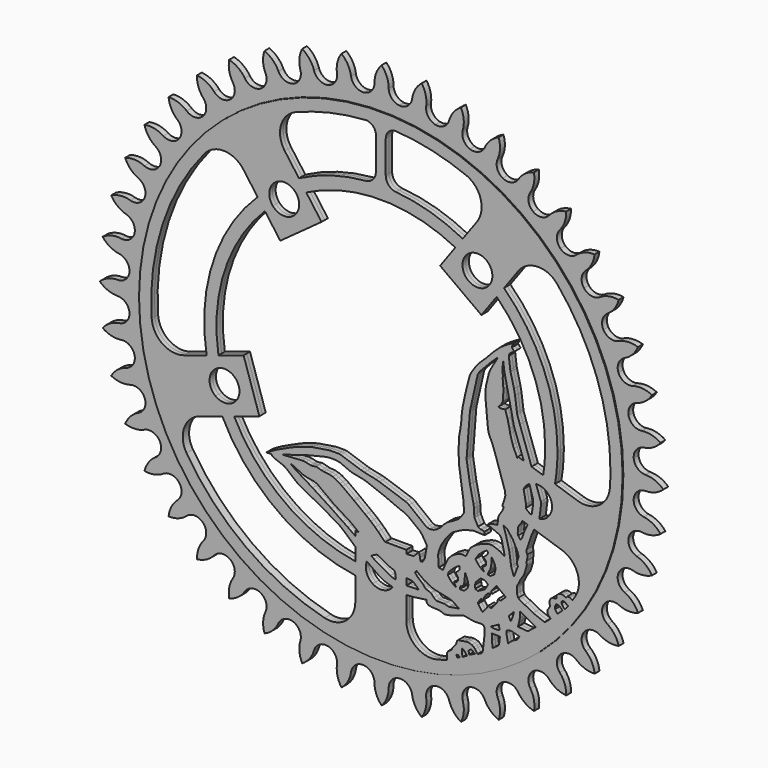
from build123d import *

# Parameters (mm, degrees)
F0_R     = 80.9142382347
F2_DEPTH = 1.016
F3_DEPTH = 1.3335


with BuildPart() as f2:
    # F0 (on Front) → F2 (new body, symmetric)
    with BuildSketch(Plane.XZ):
        with BuildLine():
            ThreePointArc((-2.3807027903, 88.3304793387), (-3.3502506643, 85.7312942415), (-5.785181868, 84.402047732))
            Line((-5.785181868, 84.402047732), (-5.784605012, 84.3980316838))
            ThreePointArc((-5.784605012, 84.3980316838), (-5.9092603745, 84.3841742706), (-6.0342913654, 84.3742627321))
            ThreePointArc((-6.0342913654, 84.3742627321), (-8.7897180441, 85.2562322534), (-10.2143039118, 87.7743270737))
            ThreePointArc((-10.2143039118, 87.7743270737), (-11.290613586, 90.8761740073), (-13.4364336422, 93.361199802))
            ThreePointArc((-13.4364336422, 93.361199802), (-14.7809344243, 90.3694083773), (-14.9266613405, 87.0926322257))
            ThreePointArc((-14.9266613405, 87.0926322257), (-15.585867257, 84.277565033), (-17.9800333254, 82.6567243326))
            ThreePointArc((-17.9800333254, 82.6567243326), (-20.8329310834, 83.1375785737), (-22.6013789781, 85.4273031122))
            ThreePointArc((-22.6013789781, 85.4273031122), (-24.1081722164, 88.3444028793), (-26.5858069626, 90.4987526602))
            ThreePointArc((-26.5858069626, 90.4987526602), (-27.4908463526, 87.346070947), (-27.1687561108, 84.0819085494))
            ThreePointArc((-27.1687561108, 84.0819085494), (-27.4206264293, 81.2016798984), (-29.5597536571, 79.2566116624))
            ThreePointArc((-29.5597536571, 79.2566116624), (-32.452045723, 79.3265618177), (-34.5283551454, 81.3413038857))
            ThreePointArc((-34.5283551454, 81.3413038857), (-36.4349579827, 84.0142727472), (-39.1939699203, 85.7940901655))
            ThreePointArc((-39.1939699203, 85.7940901655), (-39.6411239261, 82.544697672), (-38.8577733549, 79.3595979617))
            ThreePointArc((-38.8577733549, 79.3595979617), (-38.697180722, 76.4728410018), (-40.5377226476, 74.2431412103))
            ThreePointArc((-40.5377226476, 74.2431412103), (-43.4105302956, 73.9007632963), (-45.7524335735, 75.5995085554))
            ThreePointArc((-45.7524335735, 75.5995085554), (-48.0200330743, 77.9739325737), (-51.0042566765, 79.3429856792))
            ThreePointArc((-51.0042566765, 79.3429856792), (-50.9844225321, 76.063030666), (-49.7557583901, 73.0218330881))
            ThreePointArc((-49.7557583901, 73.0218330881), (-49.1859720087, 70.1873138662), (-50.6904605062, 67.7183727772))
            ThreePointArc((-50.6904605062, 67.7183727772), (-53.4853016571, 66.9706366209), (-56.0451243932, 68.3188035164))
            ThreePointArc((-56.0451243932, 68.3188035164), (-58.6275587708, 70.3463462656), (-61.776243851, 71.2767650851))
            ThreePointArc((-61.776243851, 71.2767650851), (-61.2898253223, 68.0330179777), (-59.6408596681, 65.1976325448))
            ThreePointArc((-59.6408596681, 65.1976325448), (-58.673478746, 62.4730536983), (-59.811286768, 59.8151318325))
            ThreePointArc((-59.811286768, 59.8151318325), (-62.4712665157, 58.6772591857), (-65.196898101, 59.6474029274))
            ThreePointArc((-65.196898101, 59.6474029274), (-68.0415964386, 61.286789484), (-71.2906448486, 61.7596333736))
            ThreePointArc((-71.2906448486, 61.7596333736), (-70.3475440142, 58.6181275089), (-68.3118450334, 56.0462744918))
            ThreePointArc((-68.3118450334, 56.0462744918), (-66.9665626563, 53.4871005889), (-67.7145277128, 50.6943055706))
            ThreePointArc((-67.7145277128, 50.6943055706), (-70.1854965403, 49.1894602391), (-73.0214509758, 49.7618314981))
            ThreePointArc((-73.0214509758, 49.7618314981), (-76.0705034187, 50.9796886795), (-79.3537739023, 50.9853319011))
            ThreePointArc((-79.3537739023, 50.9853319011), (-77.9731895755, 48.0100192791), (-75.5921982289, 45.7540541887))
            ThreePointArc((-75.5921982289, 45.7540541887), (-73.8964004665, 43.41238263), (-74.2392961459, 40.5415677121))
            ThreePointArc((-74.2392961459, 40.5415677121), (-76.4709522536, 38.7003840072), (-79.3594976852, 38.8633309552))
            ThreePointArc((-79.3594976852, 38.8633309552), (-82.5508343185, 39.6348667012), (-85.8014889567, 39.1731943751))
            ThreePointArc((-85.8014889567, 39.1731943751), (-84.0115258531, 36.4246437807), (-81.3337122584, 34.5304915605))
            ThreePointArc((-81.3337122584, 34.5304915605), (-79.3219206629, 32.4539920261), (-79.2527665979, 29.5635987216))
            ThreePointArc((-79.2527665979, 29.5635987216), (-81.199679903, 27.423557834), (-84.0820138756, 27.1737633411))
            ThreePointArc((-84.0820138756, 27.1737633411), (-87.3506682884, 27.4832714088), (-90.5025331271, 26.5636818521))
            ThreePointArc((-90.5025331271, 26.5636818521), (-88.3396297336, 24.0978458494), (-85.4195064533, 22.6040659762))
            ThreePointArc((-85.4195064533, 22.6040659762), (-83.1326753001, 20.8350100086), (-82.6528792681, 17.9838783899))
            ThreePointArc((-82.6528792681, 17.9838783899), (-84.2754162302, 15.5885453807), (-87.0928627361, 14.9310945424))
            ThreePointArc((-87.0928627361, 14.9310945424), (-90.3722945505, 14.7722742402), (-93.3612067107, 13.4134876445))
            ThreePointArc((-93.3612067107, 13.4134876445), (-90.8693935032, 11.2805635434), (-87.7664058264, 10.2175650679))
            ThreePointArc((-87.7664058264, 10.2175650679), (-85.2510884031, 8.791965545), (-84.3704176676, 6.0381364299))
            ThreePointArc((-84.3704176676, 6.0381364299), (-85.6355481131, 3.4362733715), (-88.3307520663, 2.384549991))
            ThreePointArc((-88.3307520663, 2.384549991), (-91.5542015078, 1.7606344421), (-94.3193153572, -0.0096882159))
            ThreePointArc((-94.3193153572, -0.0096882159), (-91.5493184668, -1.7662802314), (-88.3266342742, -2.3768577258))
            ThreePointArc((-88.3266342742, -2.3768577258), (-85.6340351899, -3.4299797088), (-84.3704176676, -6.0304463009))
            ThreePointArc((-84.3704176676, -6.0304463009), (-85.252387189, -8.7858729796), (-87.7704820093, -10.2104588474))
            ThreePointArc((-87.7704820093, -10.2104588474), (-90.8723289428, -11.2867685215), (-93.3573547375, -13.4325885778))
            ThreePointArc((-93.3573547375, -13.4325885778), (-90.3655633128, -14.7770893599), (-87.0887871612, -14.922816276))
            ThreePointArc((-87.0887871612, -14.922816276), (-84.2737199685, -15.5820221925), (-82.6528792681, -17.976188261))
            ThreePointArc((-82.6528792681, -17.976188261), (-83.1337335093, -20.8290860189), (-85.4234580477, -22.5975339137))
            ThreePointArc((-85.4234580477, -22.5975339137), (-88.3405578148, -24.1043271519), (-90.4949075957, -26.5819618981))
            ThreePointArc((-90.4949075957, -26.5819618981), (-87.3422258826, -27.4870012881), (-84.078063485, -27.1649110463))
            ThreePointArc((-84.078063485, -27.1649110463), (-81.1978348339, -27.4167813648), (-79.2527665979, -29.5559085926))
            ThreePointArc((-79.2527665979, -29.5559085926), (-79.3227167532, -32.4482006585), (-81.3374588212, -34.524510081))
            ThreePointArc((-81.3374588212, -34.524510081), (-84.0104276828, -36.4311129182), (-85.790245101, -39.1901248558))
            ThreePointArc((-85.790245101, -39.1901248558), (-82.5408526075, -39.6372788617), (-79.3557528972, -38.8539282904))
            ThreePointArc((-79.3557528972, -38.8539282904), (-76.4689959373, -38.6933356575), (-74.2392961459, -40.5338775831))
            ThreePointArc((-74.2392961459, -40.5338775831), (-73.8969182319, -43.4066852311), (-75.595663491, -45.7485885091))
            ThreePointArc((-75.595663491, -45.7485885091), (-77.9700875092, -48.0161880098), (-79.3391406147, -51.0004116121))
            ThreePointArc((-79.3391406147, -51.0004116121), (-76.0591856015, -50.9805774677), (-73.0179880236, -49.7519133256))
            ThreePointArc((-73.0179880236, -49.7519133256), (-70.1834688017, -49.1821269442), (-67.7145277128, -50.6866154417))
            ThreePointArc((-67.7145277128, -50.6866154417), (-66.9667915564, -53.4814565926), (-68.3149584519, -56.0412793287))
            ThreePointArc((-68.3149584519, -56.0412793287), (-70.3425012011, -58.6237137063), (-71.2729200207, -61.7723987865))
            ThreePointArc((-71.2729200207, -61.7723987865), (-68.0291729133, -61.2859802578), (-65.1937874804, -59.6370146037))
            ThreePointArc((-65.1937874804, -59.6370146037), (-62.4692086338, -58.6696336815), (-59.811286768, -59.8074417035))
            ThreePointArc((-59.811286768, -59.8074417035), (-58.6734141212, -62.4674214512), (-59.6435578629, -65.1930530365))
            ThreePointArc((-59.6435578629, -65.1930530365), (-61.2829444195, -68.0377513741), (-61.7557883091, -71.2867997841))
            ThreePointArc((-61.7557883091, -71.2867997841), (-58.6142824444, -70.3436989497), (-56.0424294273, -68.307999969))
            ThreePointArc((-56.0424294273, -68.307999969), (-53.4832555244, -66.9627175918), (-50.6904605062, -67.7106826483))
            ThreePointArc((-50.6904605062, -67.7106826483), (-49.1856151746, -70.1816514758), (-49.7579864336, -73.0176059113))
            ThreePointArc((-49.7579864336, -73.0176059113), (-50.975843615, -76.0666583542), (-50.9814868366, -79.3499288378))
            ThreePointArc((-50.9814868366, -79.3499288378), (-48.0061742147, -77.969344511), (-45.7502091242, -75.5883531645))
            ThreePointArc((-45.7502091242, -75.5883531645), (-43.4085375655, -73.8925554021), (-40.5377226476, -74.2354510814))
            ThreePointArc((-40.5377226476, -74.2354510814), (-38.6965389427, -76.4671071891), (-38.8594858907, -79.3556526207))
            ThreePointArc((-38.8594858907, -79.3556526207), (-39.6310216367, -82.546989254), (-39.1693493106, -85.7976438922))
            ThreePointArc((-39.1693493106, -85.7976438922), (-36.4207987163, -84.0076807886), (-34.526646496, -81.3298671939))
            ThreePointArc((-34.526646496, -81.3298671939), (-32.4501469617, -79.3180755984), (-29.5597536571, -79.2489215334))
            ThreePointArc((-29.5597536571, -79.2489215334), (-27.4197127695, -81.1958348385), (-27.1699182766, -84.0781688112))
            ThreePointArc((-27.1699182766, -84.0781688112), (-27.4794263443, -87.3468232239), (-26.5598367877, -90.4986880626))
            ThreePointArc((-26.5598367877, -90.4986880626), (-24.0940007849, -88.3357846692), (-22.6002209117, -85.4156613888))
            ThreePointArc((-22.6002209117, -85.4156613888), (-20.8311649442, -83.1288302356), (-17.9800333254, -82.6490342036))
            ThreePointArc((-17.9800333254, -82.6490342036), (-15.5847003162, -84.2715711657), (-14.9272494779, -87.0890176716))
            ThreePointArc((-14.9272494779, -87.0890176716), (-14.7684291757, -90.368449486), (-13.40964258, -93.3573616462))
            ThreePointArc((-13.40964258, -93.3573616462), (-11.2767184789, -90.8655484388), (-10.2137200034, -87.7625607619))
            ThreePointArc((-10.2137200034, -87.7625607619), (-8.7881204805, -85.2472433386), (-6.0342913654, -84.3665726031))
            ThreePointArc((-6.0342913654, -84.3665726031), (-3.4324283071, -85.6317030486), (-2.3807049265, -88.3269070018))
            ThreePointArc((-2.3807049265, -88.3269070018), (-1.7567893776, -91.5503564433), (0.0135332804, -94.3154702927))
            ThreePointArc((0.0135332804, -94.3154702927), (1.7701252959, -91.5454734023), (2.3807027903, -88.3227892097))
            ThreePointArc((2.3807027903, -88.3227892097), (3.4338247732, -85.6301901255), (6.0342913654, -84.3665726031))
            ThreePointArc((6.0342913654, -84.3665726031), (8.7897180441, -85.2485421245), (10.2143039118, -87.7666369448))
            ThreePointArc((10.2143039118, -87.7666369448), (11.290613586, -90.8684838784), (13.4364336422, -93.353509673))
            ThreePointArc((13.4364336422, -93.353509673), (14.7809344243, -90.3617182483), (14.9266613405, -87.0849420968))
            ThreePointArc((14.9266613405, -87.0849420968), (15.585867257, -84.2698749041), (17.9800333254, -82.6490342036))
            ThreePointArc((17.9800333254, -82.6490342036), (20.8329310834, -83.1298884448), (22.6013789781, -85.4196129832))
            ThreePointArc((22.6013789781, -85.4196129832), (24.1081722164, -88.3367127503), (26.5858069626, -90.4910625312))
            ThreePointArc((26.5858069626, -90.4910625312), (27.4908463526, -87.3383808181), (27.1687561108, -84.0742184205))
            ThreePointArc((27.1687561108, -84.0742184205), (27.4206264293, -81.1939897694), (29.5597536571, -79.2489215334))
            ThreePointArc((29.5597536571, -79.2489215334), (32.452045723, -79.3188716887), (34.5283551454, -81.3336137567))
            ThreePointArc((34.5283551454, -81.3336137567), (36.4349579827, -84.0065826183), (39.1939699203, -85.7864000365))
            ThreePointArc((39.1939699203, -85.7864000365), (39.6411239261, -82.537007543), (38.8577733549, -79.3519078328))
            ThreePointArc((38.8577733549, -79.3519078328), (38.697180722, -76.4651508728), (40.5377226476, -74.2354510814))
            ThreePointArc((40.5377226476, -74.2354510814), (43.4105302956, -73.8930731674), (45.7524335735, -75.5918184265))
            ThreePointArc((45.7524335735, -75.5918184265), (48.0200330743, -77.9662424447), (51.0042566765, -79.3352955502))
            ThreePointArc((51.0042566765, -79.3352955502), (50.9844225321, -76.055340537), (49.7557583901, -73.0141429592))
            ThreePointArc((49.7557583901, -73.0141429592), (49.1859720087, -70.1796237372), (50.6904605062, -67.7106826483))
            ThreePointArc((50.6904605062, -67.7106826483), (53.4853016571, -66.962946492), (56.0451243932, -68.3111133875))
            ThreePointArc((56.0451243932, -68.3111133875), (58.6275587708, -70.3386561366), (61.776243851, -71.2690749562))
            ThreePointArc((61.776243851, -71.2690749562), (61.2898253223, -68.0253278488), (59.6408596681, -65.1899424159))
            ThreePointArc((59.6408596681, -65.1899424159), (58.673478746, -62.4653635693), (59.811286768, -59.8074417035))
            ThreePointArc((59.811286768, -59.8074417035), (62.4712665157, -58.6695690567), (65.196898101, -59.6397127984))
            ThreePointArc((65.196898101, -59.6397127984), (68.0415964386, -61.2790993551), (71.2906448486, -61.7519432447))
            ThreePointArc((71.2906448486, -61.7519432447), (70.3475440142, -58.61043738), (68.3118450334, -56.0385843628))
            ThreePointArc((68.3118450334, -56.0385843628), (66.9665626563, -53.4794104599), (67.7145277128, -50.6866154417))
            ThreePointArc((67.7145277128, -50.6866154417), (70.1854965403, -49.1817701101), (73.0214509758, -49.7541413691))
            ThreePointArc((73.0214509758, -49.7541413691), (76.0705034187, -50.9719985506), (79.3537739023, -50.9776417721))
            ThreePointArc((79.3537739023, -50.9776417721), (77.9731895755, -48.0023291502), (75.5921982289, -45.7463640597))
            ThreePointArc((75.5921982289, -45.7463640597), (73.8964004665, -43.404692501), (74.2392961459, -40.5338775831))
            ThreePointArc((74.2392961459, -40.5338775831), (76.4709522536, -38.6926938782), (79.3594976852, -38.8556408262))
            ThreePointArc((79.3594976852, -38.8556408262), (82.5508343185, -39.6271765723), (85.8014889567, -39.1655042461))
            ThreePointArc((85.8014889567, -39.1655042461), (84.0115258531, -36.4169536518), (81.3337122584, -34.5228014315))
            ThreePointArc((81.3337122584, -34.5228014315), (79.3219206629, -32.4463018972), (79.2527665979, -29.5559085926))
            ThreePointArc((79.2527665979, -29.5559085926), (81.199679903, -27.415867705), (84.0820138756, -27.1660732121))
            ThreePointArc((84.0820138756, -27.1660732121), (87.3506682884, -27.4755812799), (90.5025331271, -26.5559917232))
            ThreePointArc((90.5025331271, -26.5559917232), (88.3396297336, -24.0901557204), (85.4195064533, -22.5963758473))
            ThreePointArc((85.4195064533, -22.5963758473), (83.1326753001, -20.8273198797), (82.6528792681, -17.976188261))
            ThreePointArc((82.6528792681, -17.976188261), (84.2754162302, -15.5808552517), (87.0928627361, -14.9234044134))
            ThreePointArc((87.0928627361, -14.9234044134), (90.3722945505, -14.7645841112), (93.3612067107, -13.4057975155))
            ThreePointArc((93.3612067107, -13.4057975155), (90.8693935032, -11.2728734145), (87.7664058264, -10.2098749389))
            ThreePointArc((87.7664058264, -10.2098749389), (85.2510884031, -8.7842754161), (84.3704176676, -6.0304463009))
            ThreePointArc((84.3704176676, -6.0304463009), (85.6355481131, -3.4285832426), (88.3307520663, -2.376859862))
            ThreePointArc((88.3307520663, -2.376859862), (91.5542015078, -1.7529443132), (94.3193153572, 0.0173783449))
            ThreePointArc((94.3193153572, 0.0173783449), (91.5493184668, 1.7739703604), (88.3266342742, 2.3845478548))
            ThreePointArc((88.3266342742, 2.3845478548), (85.6340351899, 3.4376698377), (84.3704176676, 6.0381364299))
            ThreePointArc((84.3704176676, 6.0381364299), (85.252387189, 8.7935631086), (87.7704820093, 10.2181489763))
            ThreePointArc((87.7704820093, 10.2181489763), (90.8723289428, 11.2944586504), (93.3573547375, 13.4402787067))
            ThreePointArc((93.3573547375, 13.4402787067), (90.3655633128, 14.7847794888), (87.0887871612, 14.930506405))
            ThreePointArc((87.0887871612, 14.930506405), (84.2737199685, 15.5897123214), (82.6528792681, 17.9838783899))
            ThreePointArc((82.6528792681, 17.9838783899), (83.1337335093, 20.8367761478), (85.4234580477, 22.6052240426))
            ThreePointArc((85.4234580477, 22.6052240426), (88.3405578148, 24.1120172809), (90.4949075957, 26.5896520271))
            ThreePointArc((90.4949075957, 26.5896520271), (87.3422258826, 27.4946914171), (84.078063485, 27.1726011753))
            ThreePointArc((84.078063485, 27.1726011753), (81.1978348339, 27.4244714937), (79.2527665979, 29.5635987216))
            ThreePointArc((79.2527665979, 29.5635987216), (79.3227167532, 32.4558907874), (81.3374588212, 34.5322002099))
            ThreePointArc((81.3374588212, 34.5322002099), (84.0104276828, 36.4388030472), (85.790245101, 39.1978149848))
            ThreePointArc((85.790245101, 39.1978149848), (82.5408526075, 39.6449689906), (79.3557528972, 38.8616184194))
            ThreePointArc((79.3557528972, 38.8616184194), (76.4689959373, 38.7010257865), (74.2392961459, 40.5415677121))
            ThreePointArc((74.2392961459, 40.5415677121), (73.8969182319, 43.4143753601), (75.595663491, 45.756278638))
            ThreePointArc((75.595663491, 45.756278638), (77.9700875092, 48.0238781388), (79.3391406147, 51.008101741))
            ThreePointArc((79.3391406147, 51.008101741), (76.0591856015, 50.9882675966), (73.0179880236, 49.7596034545))
            ThreePointArc((73.0179880236, 49.7596034545), (70.1834688017, 49.1898170732), (67.7145277128, 50.6943055706))
            ThreePointArc((67.7145277128, 50.6943055706), (66.9667915564, 53.4891467216), (68.3149584519, 56.0489694577))
            ThreePointArc((68.3149584519, 56.0489694577), (70.3425012011, 58.6314038353), (71.2729200207, 61.7800889154))
            ThreePointArc((71.2729200207, 61.7800889154), (68.0291729133, 61.2936703868), (65.1937874804, 59.6447047326))
            ThreePointArc((65.1937874804, 59.6447047326), (62.4692086338, 58.6773238104), (59.811286768, 59.8151318325))
            ThreePointArc((59.811286768, 59.8151318325), (58.6734141212, 62.4751115802), (59.6435578629, 65.2007431655))
            ThreePointArc((59.6435578629, 65.2007431655), (61.2829444195, 68.0454415031), (61.7557883091, 71.294489913))
            ThreePointArc((61.7557883091, 71.294489913), (58.6142824444, 70.3513890786), (56.0424294273, 68.3156900979))
            ThreePointArc((56.0424294273, 68.3156900979), (53.4832555244, 66.9704077208), (50.6904605062, 67.7183727772))
            ThreePointArc((50.6904605062, 67.7183727772), (49.1856151746, 70.1893416048), (49.7579864336, 73.0252960403))
            ThreePointArc((49.7579864336, 73.0252960403), (50.975843615, 76.0743484832), (50.9814868366, 79.3576189668))
            ThreePointArc((50.9814868366, 79.3576189668), (48.0061742147, 77.97703464), (45.7502091242, 75.5960432934))
            ThreePointArc((45.7502091242, 75.5960432934), (43.4085375655, 73.900245531), (40.5377226476, 74.2431412103))
            ThreePointArc((40.5377226476, 74.2431412103), (38.6965389427, 76.4747973181), (38.8594858907, 79.3633427497))
            ThreePointArc((38.8594858907, 79.3633427497), (39.6310216367, 82.5546793829), (39.1693493106, 85.8053340212))
            ThreePointArc((39.1693493106, 85.8053340212), (36.4207987163, 84.0153709176), (34.526646496, 81.3375573229))
            ThreePointArc((34.526646496, 81.3375573229), (32.4501469617, 79.3257657274), (29.5597536571, 79.2566116624))
            ThreePointArc((29.5597536571, 79.2566116624), (27.4197127695, 81.2035249675), (27.1699182766, 84.0858589401))
            ThreePointArc((27.1699182766, 84.0858589401), (27.4794263443, 87.3545133529), (26.5598367877, 90.5063781916))
            ThreePointArc((26.5598367877, 90.5063781916), (24.0940007849, 88.3434747981), (22.6002209117, 85.4233515178))
            ThreePointArc((22.6002209117, 85.4233515178), (20.8311649442, 83.1365203646), (17.9800333254, 82.6567243326))
            ThreePointArc((17.9800333254, 82.6567243326), (15.5847003162, 84.2792612946), (14.9272494779, 87.0967078006))
            ThreePointArc((14.9272494779, 87.0967078006), (14.7684291757, 90.376139615), (13.40964258, 93.3650517752))
            ThreePointArc((13.40964258, 93.3650517752), (11.2767184789, 90.8732385677), (10.2137200034, 87.7702508909))
            ThreePointArc((10.2137200034, 87.7702508909), (8.7881204805, 85.2549334675), (6.0342913654, 84.3742627321))
            ThreePointArc((6.0342913654, 84.3742627321), (5.9092603745, 84.3841742706), (5.784605012, 84.3980316838))
            Line((5.784605012, 84.3980316838), (5.785181868, 84.402047732))
            ThreePointArc((5.785181868, 84.402047732), (3.3489026704, 85.7328505084), (2.3807049265, 88.3345971308))
            ThreePointArc((2.3807049265, 88.3345971308), (1.7567893776, 91.5580465723), (-0.0135332804, 94.3231604217))
            ThreePointArc((-0.0135332804, 94.3231604217), (-1.7701252959, 91.5531635313), (-2.3807027903, 88.3304793387))
        make_face()
        with Locations((0, -0.1371763303)):
            Circle(F0_R, mode=Mode.SUBTRACT)
    extrude(amount=F2_DEPTH, both=True)

    # F0 (on Front) + F1 (on Front) → F3 (join, symmetric)
    with BuildSketch(Plane.XZ):
        with Locations((0, -0.1371763303)):
            Circle(F0_R)
        with BuildLine():
            ThreePointArc((59.0317664993, 49.1858312889), (72.2472248739, 26.1563922256), (76.835, 0.0038450645))
            ThreePointArc((76.835, 0.0038450645), (76.7927755196, -2.5430850483), (76.666148487, -5.0872158431))
            ThreePointArc((76.666148487, -5.0872158431), (73.0744274295, -23.7394756983), (65.0166675393, -40.9406315726))
            ThreePointArc((65.0166675393, -40.9406315726), (45.1624798599, -62.1569756983), (18.8492561247, -74.4832193732))
            ThreePointArc((18.8492561247, -74.4832193732), (0, -76.8311549355), (-18.8492561247, -74.4832193732))
            ThreePointArc((-18.8492561247, -74.4832193732), (-45.1624798599, -62.1569756983), (-65.0166675393, -40.9406315726))
            ThreePointArc((-65.0166675393, -40.9406315726), (-73.0744274295, -23.7394756983), (-76.666148487, -5.0872158431))
            ThreePointArc((-76.666148487, -5.0872158431), (-73.0744274295, 23.7471658273), (-59.0317664993, 49.1858312889))
            ThreePointArc((-59.0317664993, 49.1858312889), (-45.1624798599, 62.1646658273), (-28.5330294268, 71.3444608225))
            ThreePointArc((-28.5330294268, 71.3444608225), (-17.0590244353, 74.9211789086), (-5.1676308023, 76.6648704743))
            ThreePointArc((-5.1676308023, 76.6648704743), (0, 76.8388450645), (5.1676308023, 76.6648704743))
            ThreePointArc((5.1676308023, 76.6648704743), (17.0590244353, 74.9211789086), (28.5330294268, 71.3444608225))
            ThreePointArc((28.5330294268, 71.3444608225), (45.1624798599, 62.1646658273), (59.0317664993, 49.1858312889))
        make_face(mode=Mode.SUBTRACT)
        with BuildLine():
            ThreePointArc((-76.666148487, -5.0872158431), (-73.0744274295, -23.7394756983), (-65.0166675393, -40.9406315726))
            ThreePointArc((-65.0166675393, -40.9406315726), (-65.7958321334, -33.7102587401), (-60.5690531989, -28.653958637))
            Line((-60.5690531989, -28.653958637), (-53.0574761233, -26.2132992954))
            ThreePointArc((-53.0574761233, -26.2132992954), (-54.2531303783, -23.6245730703), (-55.3225672779, -20.9812045218))
            ThreePointArc((-55.3225672779, -20.9812045218), (-57.067147534, -18.5255649228), (-57.0844390827, -15.5133519302))
            ThreePointArc((-57.0844390827, -15.5133519302), (-57.7576015726, -12.7514310465), (-58.2972156627, -9.9603432049))
            Line((-58.2972156627, -9.9603432049), (-65.84602775, -12.4131009352))
            ThreePointArc((-65.84602775, -12.4131009352), (-73.0465993656, -11.3946917979), (-76.666148487, -5.0872158431))
        make_face()
        with BuildLine():
            ThreePointArc((-32.1567589923, 58.7900914961), (-33.4132933444, 65.9529477828), (-28.5330294268, 71.3444608225))
            ThreePointArc((-28.5330294268, 71.3444608225), (-45.1624798599, 62.1646658273), (-59.0317664993, 49.1858312889))
            ThreePointArc((-59.0317664993, 49.1858312889), (-52.3960484026, 52.1611689343), (-45.9720577247, 48.7526894299))
            Line((-45.9720577247, 48.7526894299), (-41.232635647, 42.2294345687))
            ThreePointArc((-41.232635647, 42.2294345687), (-39.228199606, 44.0918674886), (-37.1397367415, 45.8595617741))
            ThreePointArc((-37.1397367415, 45.8595617741), (-35.2610281077, 48.5492802232), (-32.1195407916, 49.4954244559))
            ThreePointArc((-32.1195407916, 49.4954244559), (-29.7931161901, 50.9258258254), (-27.4031144293, 52.2472610633))
            Line((-27.4031144293, 52.2472610633), (-32.1567589923, 58.7900914961))
        make_face()
        with BuildLine():
            ThreePointArc((45.9720577247, 48.7526894299), (52.3960484026, 52.1611689343), (59.0317664993, 49.1858312889))
            ThreePointArc((59.0317664993, 49.1858312889), (45.1624798599, 62.1646658273), (28.5330294268, 71.3444608225))
            ThreePointArc((28.5330294268, 71.3444608225), (33.4132933444, 65.9529477828), (32.1567589923, 58.7900914961))
            Line((32.1567589923, 58.7900914961), (27.4031144293, 52.2472610633))
            ThreePointArc((27.4031144293, 52.2472610633), (29.7931161901, 50.9258258254), (32.1195407916, 49.4954244559))
            ThreePointArc((32.1195407916, 49.4954244559), (35.2610281077, 48.5492802232), (37.1397367415, 45.8595617741))
            ThreePointArc((37.1397367415, 45.8595617741), (39.228199606, 44.0918674886), (41.232635647, 42.2294345687))
            Line((41.232635647, 42.2294345687), (45.9720577247, 48.7526894299))
        make_face()
        with BuildLine():
            ThreePointArc((65.0166675393, -40.9406315726), (73.0744274295, -23.7394756983), (76.666148487, -5.0872158431))
            ThreePointArc((76.666148487, -5.0872158431), (73.0465993656, -11.3946917979), (65.84602775, -12.4131009352))
            Line((65.84602775, -12.4131009352), (58.2972156627, -9.9603432049))
            ThreePointArc((58.2972156627, -9.9603432049), (57.7576015726, -12.7514310465), (57.0844390827, -15.5133519302))
            ThreePointArc((57.0844390827, -15.5133519302), (57.2518748466, -16.2443107258), (57.3081083962, -16.9920896261))
            ThreePointArc((57.3081083962, -16.9920896261), (56.7842839071, -19.2200601815), (55.3225672779, -20.9812045218))
            ThreePointArc((55.3225672779, -20.9812045218), (54.2531303783, -23.6245730703), (53.0574761233, -26.2132992954))
            Line((53.0574761233, -26.2132992954), (60.5690531989, -28.653958637))
            ThreePointArc((60.5690531989, -28.653958637), (65.7958321334, -33.7102587401), (65.0166675393, -40.9406315726))
        make_face()
        with BuildLine():
            ThreePointArc((4.9992490467, -54.909500628), (6.7723466361, -54.718632165), (8.5383241814, -54.4703799923))
            Line((8.5383241814, -54.4703799923), (8.5383241814, -45.5046991249))
            Line((8.5383241814, -45.5046991249), (0, -45.5046991249))
            Line((0, -45.5046991249), (-8.5383241814, -45.5046991249))
            Line((-8.5383241814, -45.5046991249), (-8.5383241814, -54.4703799923))
            ThreePointArc((-8.5383241814, -54.4703799923), (-6.7723466361, -54.718632165), (-4.9992490467, -54.909500628))
            ThreePointArc((-4.9992490467, -54.909500628), (0, -49.9961549355), (4.9992490467, -54.909500628))
        make_face()
        with BuildLine():
            Line((-8.5383241814, -54.4703799923), (-8.5383241814, -58.6363812962))
            ThreePointArc((-8.5383241814, -58.6363812962), (-5.6343782063, -58.9871019352), (-2.7166392727, -59.1937579494))
            ThreePointArc((-2.7166392727, -59.1937579494), (-4.4127597191, -57.3472295114), (-4.9992490467, -54.909500628))
            ThreePointArc((-4.9992490467, -54.909500628), (-6.7723466361, -54.718632165), (-8.5383241814, -54.4703799923))
        make_face()
        with BuildLine():
            ThreePointArc((-18.8492561247, -74.4832193732), (0, -76.8311549355), (18.8492561247, -74.4832193732))
            ThreePointArc((18.8492561247, -74.4832193732), (11.7319878261, -72.9899408568), (8.5383241814, -66.4564960314))
            Line((8.5383241814, -66.4564960314), (8.5383241814, -58.6363812962))
            ThreePointArc((8.5383241814, -58.6363812962), (5.6343782063, -58.9871019352), (2.7166392727, -59.1937579494))
            ThreePointArc((2.7166392727, -59.1937579494), (0, -59.9961549355), (-2.7166392727, -59.1937579494))
            ThreePointArc((-2.7166392727, -59.1937579494), (-5.6343782063, -58.9871019352), (-8.5383241814, -58.6363812962))
            Line((-8.5383241814, -58.6363812962), (-8.5383241814, -66.4564960314))
            ThreePointArc((-8.5383241814, -66.4564960314), (-11.7319878261, -72.9899408568), (-18.8492561247, -74.4832193732))
        make_face()
        with BuildLine():
            ThreePointArc((2.7166392727, -59.1937579494), (5.6343782063, -58.9871019352), (8.5383241814, -58.6363812962))
            Line((8.5383241814, -58.6363812962), (8.5383241814, -54.4703799923))
            ThreePointArc((8.5383241814, -54.4703799923), (6.7723466361, -54.718632165), (4.9992490467, -54.909500628))
            ThreePointArc((4.9992490467, -54.909500628), (4.9998122582, -54.9528261548), (5, -54.9961549355))
            ThreePointArc((5, -54.9961549355), (4.3922201882, -57.3853811321), (2.7166392727, -59.1937579494))
        make_face()
        with BuildLine():
            Line((-54.3336734843, -8.6725102842), (-58.2972156627, -9.9603432049))
            ThreePointArc((-58.2972156627, -9.9603432049), (-57.7576015726, -12.7514310465), (-57.0844390827, -15.5133519302))
            ThreePointArc((-57.0844390827, -15.5133519302), (-55.7985794885, -13.4120600796), (-53.6653923522, -12.1798364883))
            ThreePointArc((-53.6653923522, -12.1798364883), (-54.0280009779, -10.4315976514), (-54.3336734843, -8.6725102842))
        make_face()
        with BuildLine():
            Line((-38.7844639466, 38.8598153021), (-41.232635647, 42.2294345687))
            ThreePointArc((-41.232635647, 42.2294345687), (-56.191556763, 18.2358721381), (-58.2972156627, -9.9603432049))
            Line((-58.2972156627, -9.9603432049), (-54.3336734843, -8.6725102842))
            ThreePointArc((-54.3336734843, -8.6725102842), (-52.274060236, 16.9631928599), (-38.7844639466, 38.8598153021))
        make_face()
        with BuildLine():
            ThreePointArc((-50.6005196253, -21.6914662432), (-49.8748887134, -23.321124998), (-49.096788959, -24.9263940251))
            Line((-49.096788959, -24.9263940251), (-40.6427102229, -22.1794973302))
            Line((-40.6427102229, -22.1794973302), (-43.2811974984, -14.0590684793))
            Line((-43.2811974984, -14.0590684793), (-45.9196847739, -5.9386396284))
            Line((-45.9196847739, -5.9386396284), (-54.3336734843, -8.6725102842))
            ThreePointArc((-54.3336734843, -8.6725102842), (-54.0280009779, -10.4315976514), (-53.6653923522, -12.1798364883))
            ThreePointArc((-53.6653923522, -12.1798364883), (-49.2903625305, -13.0054607382), (-47.3081083962, -16.9920896261))
            ThreePointArc((-47.3081083962, -16.9920896261), (-48.2131148764, -19.8610664599), (-50.6005196253, -21.6914662432))
        make_face()
        with BuildLine():
            ThreePointArc((-53.0574761233, -26.2132992954), (-34.8040904981, -47.9256189296), (-8.5383241814, -58.6363812962))
            Line((-8.5383241814, -58.6363812962), (-8.5383241814, -54.4703799923))
            ThreePointArc((-8.5383241814, -54.4703799923), (-32.3830718645, -44.5931844351), (-49.096788959, -24.9263940251))
            Line((-49.096788959, -24.9263940251), (-53.0574761233, -26.2132992954))
        make_face()
        with BuildLine():
            ThreePointArc((-55.3225672779, -20.9812045218), (-54.2531303783, -23.6245730703), (-53.0574761233, -26.2132992954))
            Line((-53.0574761233, -26.2132992954), (-49.096788959, -24.9263940251))
            ThreePointArc((-49.096788959, -24.9263940251), (-49.8748887134, -23.321124998), (-50.6005196253, -21.6914662432))
            ThreePointArc((-50.6005196253, -21.6914662432), (-53.0518121678, -21.9364707502), (-55.3225672779, -20.9812045218))
        make_face()
        with BuildLine():
            ThreePointArc((-37.1397367415, 45.8595617741), (-39.228199606, 44.0918674886), (-41.232635647, 42.2294345687))
            Line((-41.232635647, 42.2294345687), (-38.7844639466, 38.8598153021))
            ThreePointArc((-38.7844639466, 38.8598153021), (-37.4962240555, 40.1000350739), (-36.1683471587, 41.2977203609))
            ThreePointArc((-36.1683471587, 41.2977203609), (-37.2185471541, 43.4584364341), (-37.1397367415, 45.8595617741))
        make_face()
        with BuildLine():
            ThreePointArc((-28.0881850893, 47.1497548282), (-26.5350623242, 48.0384447602), (-24.9538522165, 48.8761408351))
            Line((-24.9538522165, 48.8761408351), (-27.4031144293, 52.2472610633))
            ThreePointArc((-27.4031144293, 52.2472610633), (-29.7931161901, 50.9258258254), (-32.1195407916, 49.4954244559))
            ThreePointArc((-32.1195407916, 49.4954244559), (-29.8135979812, 48.8214498757), (-28.0881850893, 47.1497548282))
        make_face()
        with BuildLine():
            Line((-19.8416017616, 41.839731736), (-24.9538522165, 48.8761408351))
            ThreePointArc((-24.9538522165, 48.8761408351), (-26.5350623242, 48.0384447602), (-28.0881850893, 47.1497548282))
            ThreePointArc((-28.0881850893, 47.1497548282), (-27.5219419549, 45.8781811963), (-27.3281888761, 44.4997797551))
            ThreePointArc((-27.3281888761, 44.4997797551), (-30.6253664269, 39.798673959), (-36.1683471587, 41.2977203609))
            ThreePointArc((-36.1683471587, 41.2977203609), (-37.4962240555, 40.1000350739), (-38.7844639466, 38.8598153021))
            Line((-38.7844639466, 38.8598153021), (-33.656900494, 31.8023296698))
            Line((-33.656900494, 31.8023296698), (-26.7492511278, 36.8210307029))
            Line((-26.7492511278, 36.8210307029), (-19.8416017616, 41.839731736))
        make_face()
        with BuildLine():
            ThreePointArc((1.651, 73.3773110308), (2.6958039071, 75.7843184723), (5.1676308023, 76.6648704743))
            ThreePointArc((5.1676308023, 76.6648704743), (0, 76.8388450645), (-5.1676308023, 76.6648704743))
            ThreePointArc((-5.1676308023, 76.6648704743), (-2.6958039071, 75.7843184723), (-1.651, 73.3773110308))
            Line((-1.651, 73.3773110308), (-1.651, 62.5100089261))
            ThreePointArc((-1.651, 62.5100089261), (-2.640616689, 59.9672529237), (-5.0887527253, 58.7624379059))
            ThreePointArc((-5.0887527253, 58.7624379059), (0, 58.9818558122), (5.0887527253, 58.7624379059))
            ThreePointArc((5.0887527253, 58.7624379059), (2.640616689, 59.9672529237), (1.651, 62.5100089261))
            Line((1.651, 62.5100089261), (1.651, 73.3773110308))
        make_face()
        with BuildLine():
            Line((24.9538522165, 48.8761408351), (27.4031144293, 52.2472610633))
            ThreePointArc((27.4031144293, 52.2472610633), (16.5693162237, 56.6124291428), (5.0887527253, 58.7624379059))
            ThreePointArc((5.0887527253, 58.7624379059), (0, 58.9818558122), (-5.0887527253, 58.7624379059))
            ThreePointArc((-5.0887527253, 58.7624379059), (-16.5693162237, 56.6124291428), (-27.4031144293, 52.2472610633))
            Line((-27.4031144293, 52.2472610633), (-24.9538522165, 48.8761408351))
            ThreePointArc((-24.9538522165, 48.8761408351), (0, 54.8628236697), (24.9538522165, 48.8761408351))
        make_face()
        with BuildLine():
            ThreePointArc((32.1195407916, 49.4954244559), (29.7931161901, 50.9258258254), (27.4031144293, 52.2472610633))
            Line((27.4031144293, 52.2472610633), (24.9538522165, 48.8761408351))
            ThreePointArc((24.9538522165, 48.8761408351), (26.5350623242, 48.0384447602), (28.0881850893, 47.1497548282))
            ThreePointArc((28.0881850893, 47.1497548282), (29.8135979812, 48.8214498757), (32.1195407916, 49.4954244559))
        make_face()
        with BuildLine():
            Line((38.7844639466, 38.8598153021), (41.232635647, 42.2294345687))
            ThreePointArc((41.232635647, 42.2294345687), (39.228199606, 44.0918674886), (37.1397367415, 45.8595617741))
            ThreePointArc((37.1397367415, 45.8595617741), (37.2808517622, 45.1861691027), (37.3281888761, 44.4997797551))
            ThreePointArc((37.3281888761, 44.4997797551), (37.0292946722, 42.7969573059), (36.1683471587, 41.2977203609))
            ThreePointArc((36.1683471587, 41.2977203609), (37.4962240555, 40.1000350739), (38.7844639466, 38.8598153021))
        make_face()
        with BuildLine():
            ThreePointArc((59.1190321425, -0.1371763303), (54.4641784736, 22.8565885782), (41.232635647, 42.2294345687))
            Line((41.232635647, 42.2294345687), (38.7844639466, 38.8598153021))
            ThreePointArc((38.7844639466, 38.8598153021), (50.7845720523, 20.9798130732), (55, -0.1371763303))
            ThreePointArc((55, -0.1371763303), (54.8331653365, -4.4178280544), (54.3336734843, -8.6725102842))
            Line((54.3336734843, -8.6725102842), (58.2972156627, -9.9603432049))
            ThreePointArc((58.2972156627, -9.9603432049), (58.913219773, -5.065918304), (59.1190321425, -0.1371763303))
        make_face()
        with BuildLine():
            ThreePointArc((57.0844390827, -15.5133519302), (57.7576015726, -12.7514310465), (58.2972156627, -9.9603432049))
            Line((58.2972156627, -9.9603432049), (54.3336734843, -8.6725102842))
            ThreePointArc((54.3336734843, -8.6725102842), (54.0280009779, -10.4315976514), (53.6653923522, -12.1798364883))
            ThreePointArc((53.6653923522, -12.1798364883), (55.7985794885, -13.4120600796), (57.0844390827, -15.5133519302))
        make_face()
        with BuildLine():
            Line((49.096788959, -24.9263940251), (53.0574761233, -26.2132992954))
            ThreePointArc((53.0574761233, -26.2132992954), (54.2531303783, -23.6245730703), (55.3225672779, -20.9812045218))
            ThreePointArc((55.3225672779, -20.9812045218), (53.0518121678, -21.9364707502), (50.6005196253, -21.6914662432))
            ThreePointArc((50.6005196253, -21.6914662432), (49.8748887134, -23.321124998), (49.096788959, -24.9263940251))
        make_face()
        with BuildLine():
            ThreePointArc((53.6653923522, -12.1798364883), (54.0280009779, -10.4315976514), (54.3336734843, -8.6725102842))
            Line((54.3336734843, -8.6725102842), (45.9196847739, -5.9386396284))
            Line((45.9196847739, -5.9386396284), (43.2811974984, -14.0590684793))
            Line((43.2811974984, -14.0590684793), (40.6427102229, -22.1794973302))
            Line((40.6427102229, -22.1794973302), (49.096788959, -24.9263940251))
            ThreePointArc((49.096788959, -24.9263940251), (49.8748887134, -23.321124998), (50.6005196253, -21.6914662432))
            ThreePointArc((50.6005196253, -21.6914662432), (47.5490692585, -15.4586143295), (53.6653923522, -12.1798364883))
        make_face()
        with BuildLine():
            Line((33.656900494, 31.8023296698), (38.7844639466, 38.8598153021))
            ThreePointArc((38.7844639466, 38.8598153021), (37.4962240555, 40.1000350739), (36.1683471587, 41.2977203609))
            ThreePointArc((36.1683471587, 41.2977203609), (29.3953496445, 40.450279287), (28.0881850893, 47.1497548282))
            ThreePointArc((28.0881850893, 47.1497548282), (26.5350623242, 48.0384447602), (24.9538522165, 48.8761408351))
            Line((24.9538522165, 48.8761408351), (19.8416017616, 41.839731736))
            Line((19.8416017616, 41.839731736), (26.7492511278, 36.8210307029))
            Line((26.7492511278, 36.8210307029), (33.656900494, 31.8023296698))
        make_face()
    with BuildSketch(Plane.XZ):
        Polygon((46.6831956419, -61.5737032045), (47.5812781038, -60.8994206753), (48.6355330585, -59.9776573462), (53.4171865707, -56.1212764749), (57.4362192418, -52.8593834472), (58.5288416104, -51.7090210453), (62.8087746777, -47.0545024943), (65.9125627449, -43.6881482804), (66.058076278, -43.5004226158), (65.670976248, -43.2249680536), (64.5092297934, -42.4406144534), (63.3138863773, -41.7788137834), (63.0730180895, -41.742376387), (62.3480545223, -41.7782593777), (62.1221604324, -42.2489481377), (61.168764779, -41.8628117287), (60.6291599421, -41.7480191783), (60.1618625187, -41.7477183594), (59.4649632789, -42.0041282935), (59.3255420286, -42.1287008646), (58.8413912477, -42.599283044), (58.7685374338, -43.2434126629), (58.7416268465, -43.4877907459), (58.3100764388, -43.6235148822), (57.2308070672, -43.9258016386), (56.8557707955, -44.2204479187), (56.5171714784, -44.9215208599), (56.4836567768, -45.2245601561), (56.5641248133, -46.4690712594), (56.5754614335, -46.6558013338), (56.0642236365, -47.4727083795), (55.7486515521, -47.8189317854), (55.8094915439, -48.7072010587), (56.0927093422, -49.364728291), (56.5401679052, -49.8944570802), (56.8629870697, -50.1140840112), (56.6848119853, -50.3019512254), (55.0419831128, -51.6911684081), (54.7400271363, -51.7828404447), (50.9291490158, -50.3210445196), (48.107756603, -48.793802106), (46.4195525156, -47.9217788388), (45.9842437131, -47.5422810436), (45.948467544, -47.4912532747), (45.5946027635, -46.4291886705), (45.5514050364, -44.6217471454), (45.665805089, -43.9860189658), (46.8932164308, -41.6076725186), (47.7842523129, -40.3327358386), (47.9898784126, -39.9201745856), (48.8175623107, -37.2389904639), (48.8571946987, -36.7197324434), (48.7752955483, -35.9486336497), (48.9930694632, -35.3179268578), (49.0456909211, -33.7480829907), (48.8352167601, -33.3660885177), (48.7608766937, -32.5938004166), (50.4458389016, -27.5359156545), (51.3126889758, -25.574369393), (52.7177806174, -23.0773786634), (53.0282541924, -22.137425494), (53.6261615429, -17.5294067059), (53.5263739358, -16.54977559), (51.9771325269, -12.1078309864), (51.248487621, -9.6923367221), (46.5288804707, 3.7718431503), (45.6836971359, 6.314066246), (45.5763672041, 6.8952757488), (44.9214814151, 11.7765993171), (44.5589530035, 13.6724199563), (43.4208974614, 18.2382447717), (43.3162293155, 18.8198923772), (42.8198484588, 22.747465594), (43.169372095, 23.6395642115), (43.3592487176, 23.800848521), (44.5532069566, 24.5611327942), (44.673540364, 24.6176063223), (44.625979234, 24.6956744861), (43.858434909, 25.5490268028), (43.8359746193, 25.7507457739), (44.354245494, 26.9452772123), (44.279325213, 27.0450641525), (41.9135512722, 25.6581482321), (40.0703419751, 24.434330377), (37.8356473631, 22.4068626254), (35.2206709969, 19.6481969356), (32.9593875977, 17.4584472616), (31.735291218, 16.0160176612), (30.1093418296, 13.5074232273), (29.7154530301, 12.5647860203), (28.4810972733, 7.7321556873), (27.8173170201, 4.7821822271), (27.4116715759, 2.8594510986), (27.1030622503, 0.637751111), (26.866428754, -2.4096343835), (26.4652813958, -4.8705677033), (26.1371624018, -6.7438038627), (26.1119450172, -7.9570074089), (26.0283647529, -11.0410313597), (26.1758514529, -14.7372823439), (27.6590966053, -24.9169858249), (27.8402649705, -28.0277747248), (27.7734176965, -28.3607163634), (27.6171860348, -28.6954924287), (26.5055345609, -30.3119348483), (25.9166566291, -30.855620111), (24.1595617086, -31.9262969432), (22.4317592546, -32.8550922818), (21.3766469356, -33.706957472), (19.9256328236, -35.2870546544), (18.831429982, -36.1135260291), (18.5772070523, -36.294059763), (17.6660786287, -36.6725642412), (16.2486361804, -36.8857952572), (15.3465713423, -36.6490794428), (9.4334289916, -32.020445214), (8.2366649026, -31.3662777573), (-0.441770063, -28.4106707478), (-1.7034291822, -28.0639884495), (-5.5176427354, -27.2551771538), (-6.6285873458, -26.9469542464), (-13.3378052521, -24.689769201), (-14.0037068978, -24.5405497327), (-17.3119494391, -24.6061987738), (-22.849807139, -25.4937548426), (-23.6977238108, -25.6887872926), (-28.1716458426, -27.1326565287), (-30.8872106853, -28.3036820205), (-35.1480155009, -30.2951713538), (-36.8980466944, -31.2504734299), (-37.868184967, -31.8142363175), (-37.9840150293, -31.8317652281), (-38.3066577344, -32.077386975), (-38.2958091795, -32.1438796818), (-38.1569601796, -32.0794210143), (-36.7569361732, -32.0060480911), (-36.5777517753, -32.1030363054), (-36.3733950131, -32.3777320093), (-35.6317629028, -32.9085575926), (-32.3990644655, -34.1206189058), (-31.3362430876, -34.8762610982), (-28.3060470111, -37.4205235853), (-27.3723523848, -38.037433165), (-20.3260205967, -41.8448480332), (-14.2797610993, -45.27028905), (-12.958210906, -46.2570086067), (-10.0057958183, -48.8410748108), (-7.1521555829, -51.445988683), (-6.3267229571, -52.0562156278), (-0.0023595678, -56.5484602559), (1.0200355028, -57.0668506977), (5.0013280915, -58.3342531477), (7.8452084183, -58.8409668424), (10.6699476084, -58.6840698024), (14.8066808068, -58.1163415838), (15.2528321894, -58.0645776734), (15.3585449644, -58.7568125718), (15.8362714574, -59.3838347928), (17.0401656957, -59.6469117761), (19.3151648986, -59.7261136802), (19.769207262, -59.813279803), (21.2148599963, -60.3074324644), (21.4851240846, -60.3627592051), (22.7767529719, -60.1651904988), (24.2517543137, -59.7761124421), (26.5477541765, -58.996295574), (27.5242401355, -58.6845781715), (28.2326878168, -58.7034204588), (30.7747326531, -59.1921645607), (31.5479414991, -59.2504150334), (33.7903648038, -59.152266797), (34.3090327519, -59.2983175269), (34.7808940467, -60.1270004714), (34.7467235174, -61.8667252237), (34.0682898332, -67.3447117468), (33.8751106273, -67.6760856806), (33.6009251534, -67.8818147802), (32.3918120193, -68.4514091185), (31.5252445966, -67.2973940106), (31.102840748, -66.7972256344), (30.491067291, -66.3926853081), (29.1369765865, -66.0267196893), (28.4006910206, -66.046137301), (28.1646121747, -66.1229368873), (26.9501682828, -66.35533207), (25.8987841228, -66.4684873644), (25.5262142926, -66.7872880461), (25.1913481464, -67.9544501162), (24.6811797251, -68.5655603057), (23.9200117233, -69.437873978), (23.7594467905, -69.9403277494), (23.2888612485, -70.381350486), (22.6102866381, -70.764175726), (22.1181994204, -71.4731471217), (22.0721975074, -71.7180757268), (22.0737613507, -74.5819409526), (22.1672718947, -75.3458172404), (22.3442650865, -75.306617694), (30.34654073, -71.8449526537), (31.8908199225, -71.0367179174), (35.3018348643, -69.1563670634), (39.1357467304, -66.7719095835), (44.4581563277, -63.0650203976), (46.3333588474, -61.7747918264), align=None)
        Polygon((12.5345016562, -55.7321072872), (12.7065571754, -55.9188380392), (12.1483366793, -55.961446431), (7.6905966583, -56.0520908348), (6.060515984, -55.8202617107), (3.9652106983, -55.2101355764), (3.166212467, -54.8660649398), (-2.2208206177, -51.7935426326), (-5.5278550457, -49.7361127025), (-6.6220127744, -48.7667562506), (-8.6913856385, -46.8778741883), (-11.0341272198, -45.2260306279), (-12.7806391415, -44.0837600164), (-16.5562533499, -41.4928894848), (-22.8736538387, -37.4383028846), (-28.6729240125, -33.9003690987), (-30.1666653409, -32.7868348983), (-29.6095420649, -32.9160411461), (-26.1201132177, -34.5782872106), (-24.9970376774, -34.9392969705), (-22.293139425, -35.409895821), (-21.2443662824, -35.8619304218), (-15.9562942011, -39.7674841304), (-13.6456192222, -41.2415301542), (-10.0760823642, -43.4672598908), (-8.217554636, -44.8794383194), (-6.0132016154, -46.6621657978), (-4.6950732825, -47.546129337), (-4.518647706, -47.6165820481), (-3.0980649763, -45.5802983971), (-3.0827190668, -45.8797459307), (-2.8802347866, -48.6443169118), (-2.4062962859, -49.2656011169), (0.9658814178, -51.3370563478), (2.035960168, -51.9089120882), (2.884095837, -52.3024958547), (6.1560690639, -53.49378164), (6.5539917552, -53.5624880771), (7.5495364805, -53.6324058837), (10.4135749987, -54.0494119457), (11.1461064991, -54.4346738869), align=None, mode=Mode.SUBTRACT)
        Polygon((-32.6622608318, -30.9599802131), (-32.675752719, -30.889360667), (-32.1535107866, -30.7053098312), (-24.2520735911, -28.3288506818), (-20.8349917476, -27.490434755), (-18.1382455722, -26.8510619843), (-16.9668776492, -26.7295471057), (-14.8160007083, -26.7767854152), (-13.638531738, -27.0345415447), (-10.4873480973, -28.3862130977), (-9.3597342095, -28.7359485759), (-5.903819532, -29.4262139772), (-4.9171079528, -29.7095131175), (1.1423046444, -32.0190345571), (1.5147972447, -32.177700897), (6.2160083619, -34.1754453047), (8.1214368301, -34.8654564514), (9.2122036458, -35.5087703203), (13.0889984055, -38.5315105495), (13.8037053943, -39.3391678777), (14.6288550026, -40.694425225), (14.7280138239, -40.8138528478), (15.3879051283, -42.0162853952), (15.3907488917, -42.2892960138), (14.7519890123, -45.8500945087), (14.6727230509, -46.1166170358), (13.9245380202, -47.3848149534), (13.3490067793, -47.3314542667), (13.0704140853, -46.4468010713), (12.9999895939, -45.4831581408), (12.6670954724, -44.9012221618), (12.0348100164, -45.5581171582), (11.316362418, -46.3358763217), (10.769375647, -46.5875923686), (8.5346914483, -46.7516421947), (6.4190596883, -46.7946445929), (5.4623141118, -46.66867986), (1.990439042, -45.7986017469), (1.0953286761, -45.2539521896), (-0.8805950684, -43.2193602517), (-1.9308215018, -42.2455618925), (-3.3593218899, -40.9919578756), (-5.1504187575, -39.5936475962), (-8.8156751726, -36.7977559799), (-9.1661537421, -36.5386914176), (-12.8830547392, -33.8126521044), (-13.744970248, -33.2534172357), (-15.1249929448, -32.4048714975), (-16.0937921701, -31.9918109345), (-17.3279190691, -31.6596307791), (-19.1444473011, -31.483071706), (-19.9118386891, -31.312462676), (-21.5437219805, -30.8506617053), (-21.8507713283, -30.885238306), (-23.2347866196, -31.0705114468), (-23.6341594656, -31.01277615), (-25.1495935383, -30.6457183338), (-26.3857678457, -30.538468739), (-32.3257866021, -30.940175144), align=None, mode=Mode.SUBTRACT)
        Polygon((25.5088127801, -71.7200132889), (25.3252056857, -70.9481036364), (25.8957612875, -70.8496178818), (26.4044579587, -71.3821956112), align=None, mode=Mode.SUBTRACT)
        Polygon((28.0504848489, -69.0925828476), (28.8172274032, -70.1261100298), (27.3726279261, -71.0151521687), (27.0981085875, -69.7603630053), (27.2342883386, -68.466514277), align=None, mode=Mode.SUBTRACT)
        Polygon((31.5836571708, -68.7033840261), (29.6013288615, -69.5669867856), (29.3331364126, -68.4224598504), (30.0296952374, -67.9080638153), (30.3221338446, -67.8717789664), align=None, mode=Mode.SUBTRACT)
        Polygon((37.2001642955, -62.9860682102), (37.1167186919, -60.8433275801), (39.8530524636, -60.8937592156), (39.8326331964, -61.1838456819), (39.5837852041, -63.286493993), (39.443554273, -63.6163433631), (37.4117975857, -65.1397758177), align=None, mode=Mode.SUBTRACT)
        Polygon((12.5312108522, -52.5020708918), (11.4226560085, -51.3192202506), (11.9096417755, -50.6184350772), (12.3035526209, -50.893522196), (14.26027202, -52.3844394938), (14.5754890058, -52.5820775436), (17.4811226675, -54.0142138099), (17.8904485241, -54.1562132746), (23.0728691972, -55.2610323707), (23.8756212191, -55.5847304589), (25.8502880335, -56.8318877855), (26.132499416, -57.0279102185), (25.9416632014, -57.1429737794), (24.7339834268, -57.3448043583), (23.1858853591, -57.6212836119), (22.6166673951, -57.6516690378), (21.5126895019, -57.3226767903), (21.1166251012, -57.2683089023), (18.7795366879, -57.2905968379), (18.3771966332, -57.1650025874), (17.795343315, -56.6259113733), (16.8150115377, -55.5837071288), (16.624689154, -55.4843537793), (15.1484226796, -54.9890002123), (14.7169324318, -54.6747717124), (14.2807197467, -53.9929801845), (13.9766352979, -53.6858196336), align=None, mode=Mode.SUBTRACT)
        Polygon((36.6985420271, -58.9763496964), (39.546829406, -57.4538706488), (39.7225243838, -59.078678048), (38.1957097669, -59.209016543), align=None, mode=Mode.SUBTRACT)
        Polygon((36.7213766867, -49.2127272662), (37.2959836279, -49.1468282663), (36.9070191273, -48.4399001541), (37.801845576, -47.3580092995), (38.6798680656, -46.2963417159), (40.1865326086, -47.4260493158), (41.7953911951, -48.6324660265), (41.1796387437, -49.2274711838), (40.3223719428, -50.0872208359), (39.9756826564, -50.2617605238), (39.2101123237, -50.0329606678), (39.0276431, -50.8090616718), (38.8005271154, -51.3099898375), (37.6689987992, -52.794485757), (37.0588112098, -53.413009418), (36.4896346055, -53.4631935276), (35.9039450466, -53.1282056379), (35.5846662597, -53.6877973471), (35.3956622647, -53.9689652785), (34.2054879497, -55.4764927424), (34.0869049279, -55.6409431828), (33.7705750919, -55.3011064976), (32.5710756221, -53.5925554235), (32.5663527588, -53.1026334878), (33.5727179848, -51.7868131694), (34.1992172686, -51.9918823024), (34.2587683103, -51.8683073954), (34.6499687782, -50.9351653802), (35.2135740454, -50.0994206006), (35.9354855313, -49.4455159478), align=None, mode=Mode.SUBTRACT)
        Polygon((46.1099289755, -58.6801942583), (46.4685303252, -58.8005285359), (45.5549667586, -59.9652736957), (45.3759130537, -60.0823485128), (44.070982449, -60.7417621153), (43.1110424221, -61.5636516218), (42.6399868575, -62.0411108718), (42.6001980881, -61.9924456177), (42.0278116821, -59.3552171447), (42.043556591, -58.5279060347), (42.0929032631, -58.4178439912), (42.7755632325, -58.0731062841), (43.5836679642, -58.0273332502), (43.949440353, -58.0792834453), align=None, mode=Mode.SUBTRACT)
        Polygon((43.5810762358, -55.1665153066), (43.515120451, -55.2307285824), (42.7871496351, -53.8447042369), (44.5169992, -52.1232629526), (44.3158547349, -53.0824907677), align=None, mode=Mode.SUBTRACT)
        Polygon((46.5009437008, -51.6328711901), (46.5106603414, -51.1959532898), (51.8131590302, -54.0963929647), (51.8878719069, -54.1770260122), (51.7021773991, -54.3420620258), (49.3448200323, -56.182773668), (48.9747072144, -56.3048130598), (46.0265492578, -56.0378898436), (45.9120353591, -56.0062540675), (46.008733945, -55.5869897242), (46.3965733436, -54.1428785518), (46.5177777416, -53.1903572018), align=None, mode=Mode.SUBTRACT)
        Polygon((25.8694998456, -44.6903117338), (26.2194048971, -44.4803947679), (26.4257640863, -45.0501878928), (26.2464271562, -45.7701043042), (25.2656120197, -46.6828248473), (25.0232258204, -46.9304746894), (25.7834549131, -47.9359293209), (25.9197855757, -48.4754052356), (25.8042768846, -49.1189224455), (25.3545224978, -49.5860450696), (24.4895219348, -49.7826564607), (25.1529472161, -51.1441943281), (24.4094499857, -50.6870013355), (23.2235475128, -49.6183969032), (22.3942699024, -48.445811764), (22.7982972271, -47.3411506434), (23.8183522228, -46.299104863), (24.3787965666, -45.7676004186), align=None, mode=Mode.SUBTRACT)
        Polygon((28.1709996849, -46.0154042495), (28.2689236404, -46.0182759499), (28.9798784858, -47.7002185615), (29.0979551529, -47.9875511187), (29.3405436767, -49.1872551321), (29.0326764554, -50.2213443981), (27.8760930322, -51.2906730905), (27.7573063173, -51.3216695499), (26.4240918798, -51.2924791668), (26.6490197485, -50.3373049472), (27.1312377013, -50.2338212809), (27.4232507126, -50.0369425335), (27.808022625, -49.3626427697), (27.9528328117, -48.797379872), (28.1974049851, -46.2248888595), align=None, mode=Mode.SUBTRACT)
        Polygon((35.2575133912, -46.3027468117), (35.8916785293, -46.9374043917), (34.7899195984, -48.682366939), (33.8987306201, -49.1527213483), (33.230224168, -49.4997706501), (32.4289477503, -49.8628289827), (31.7551447267, -49.6151919626), (31.6289972672, -49.4868355029), (31.4447420301, -48.4246630272), (31.8541084205, -47.4100707948), (32.5556729079, -46.6603961933), (33.3031312235, -45.9616297833), (33.9360301381, -45.811005242), (34.6628480791, -45.9843803003), align=None, mode=Mode.SUBTRACT)
        Polygon((32.5062463263, -41.9156785723), (31.6689629391, -40.7046335676), (32.7563418892, -39.0226100005), (34.2103751642, -37.7938654911), (35.5333917003, -36.8769346578), (35.8982080335, -37.4161788888), (35.9029001858, -37.5627118527), (35.5203294994, -38.2306778124), (34.3355771701, -39.3416356811), (34.9751092646, -39.8978859706), (35.2314176358, -40.3969541906), (35.282758722, -41.1740270009), (35.1342501023, -41.5231594015), (34.6313969493, -41.9417275896), (34.3506238717, -42.0559846472), (33.8363111588, -42.1496270318), (34.505753005, -43.5030717934), (33.6359811918, -42.973726188), align=None, mode=Mode.SUBTRACT)
        Polygon((37.097129458, -38.4848910207), (37.1731456373, -38.4710532131), (38.1077385612, -40.1085522949), (38.3270172435, -40.9708376163), (38.3502856687, -41.6529347287), (38.0222148846, -43.1339610146), (37.8597852887, -43.3463501584), (36.8080829857, -44.0145868489), (36.5783618204, -44.0793313336), (35.7809331544, -43.9973951602), (36.0285411522, -43.1860410651), (36.7179774354, -42.0243017455), (37.1018770443, -39.8129095923), (37.0870050205, -38.816139782), align=None, mode=Mode.SUBTRACT)
        Polygon((59.6104474543, -45.3645822083), (60.8425865807, -46.3619333191), (59.112459776, -47.9687003141), (58.958676036, -47.8054399483), (58.2960282302, -46.8240492943), (58.2455283854, -46.2069982527), (58.6840556919, -45.1993788277), (59.4398776029, -45.2968196972), align=None, mode=Mode.SUBTRACT)
        Polygon((62.6904354755, -44.4733590864), (62.7957326592, -44.5788807908), (61.4842310918, -45.8273924259), (60.8159076805, -44.9511021176), (60.5017545731, -44.415429751), (60.4825367378, -44.0075176658), (60.5165888849, -43.920901647), (60.7871909658, -43.5003210042), (61.4693920305, -43.6187734024), align=None, mode=Mode.SUBTRACT)
        Polygon((45.5346393246, -37.4854872599), (45.8848233119, -38.2645071425), (44.5522408799, -41.7146684636), (44.4298125474, -41.45790967), (43.7118575431, -39.367008853), (43.6082428346, -38.913106027), (42.9228219876, -34.3256279693), (41.8917528001, -30.4819642223), (41.1811954319, -28.2576887097), (41.0523926493, -27.7777714208), (42.2268304166, -28.3696426504), (42.4176834624, -28.5709320219), (42.7284944927, -29.0377265763), (43.6719977464, -30.1868356983), (44.2456592882, -30.9530651051), (44.9773009108, -32.5014078307), (45.2753747773, -32.9295889714), (45.7774350803, -34.0859021021), (46.0754018604, -35.1156873276), (46.1119365052, -35.4895978932), (45.5423896106, -37.0060301895), align=None, mode=Mode.SUBTRACT)
        Polygon((21.2863245577, -46.2829145181), (20.7965614131, -47.5286646295), (19.4089970845, -47.201419336), (19.3729066328, -46.8217789802), (19.1655792573, -43.6166581056), (19.3114774529, -42.6388349762), (20.0294035136, -40.7439154382), (20.4148384266, -39.9634676556), (21.725777294, -37.8822044793), (22.9370021311, -36.422977544), (23.8230949433, -35.5052415701), (24.2229967115, -35.2159169445), (26.8381782769, -33.829184937), (28.5207012568, -33.1752030627), (31.1157818308, -32.5769876747), (31.4577843674, -32.5702610546), (33.8866273648, -32.706897968), (34.7758409311, -32.6827329286), (34.679207505, -31.6895509746), (33.9283599192, -31.4173195099), (33.4007150784, -31.3666898363), (32.5213563043, -30.8989601435), (31.3754992857, -28.6776013121), (31.2547789888, -27.8184265304), (31.1897852249, -25.9486157167), (31.02797301, -24.8114690806), (29.8490587406, -19.328134608), (28.7364662653, -12.4680386002), (28.7303024535, -11.7842169575), (29.8070897055, 1.9612227873), (29.9752741362, 2.9750880895), (32.4328901022, 13.8361058078), (32.9449189573, 14.8135449858), (36.6078665062, 18.682287242), (38.6089827334, 20.6033002275), (39.0311175837, 20.9916921827), (39.0892248177, 20.950148893), (38.929127164, 20.6312597196), (36.7161464588, 16.8379541284), (36.1269316072, 15.3706653474), (35.2160178086, 11.5156165402), (35.1138785886, 10.776616957), (35.0133630615, 8.2522096803), (35.0572280988, 7.413480447), (35.8860151919, -1.2094075168), (36.1795045796, -2.4097093074), (37.3945207668, -5.0744965878), (38.2984654071, -7.5954870169), (41.5674048916, -17.5419613246), (41.6641434839, -18.7399932702), (41.0633987097, -22.5607238371), (40.6180139639, -23.6804423912), (39.6020290202, -25.1358568366), (39.229329672, -26.1746067096), (39.0899225984, -27.9471822927), (39.0577637467, -28.2986154163), (37.4996831865, -28.494168429), (35.7169149266, -29.2012444112), (36.1978968173, -29.4244816046), (39.695413042, -30.9195471627), (40.3564170812, -31.7170727465), (41.3589404254, -36.1239431952), (41.4652517783, -36.7668370012), (41.0937955917, -36.5609714309), (39.9032054244, -35.8203790416), (39.0010491662, -35.4055893132), (37.3656541984, -34.8888861738), (36.3529775619, -34.8485400394), (34.8948228608, -35.179003617), (33.0291565105, -35.9440936807), (31.8715575116, -36.5543300258), (31.0653634635, -37.0810837468), (30.106012503, -37.8756145515), (29.3860162255, -38.9585490856), (28.5454933032, -40.8355733885), (28.4790208464, -40.9263758416), (27.0287044404, -40.8070283686), (25.8611934597, -41.0483317506), (23.8181953297, -42.2463495613), (22.5364453592, -43.538384356), align=None, mode=Mode.SUBTRACT)
        Polygon((47.1898538564, -11.7317632395), (47.0862970438, -11.2691048641), (45.5517839646, -11.3316908191), (46.3267748857, -10.364608707), (46.5769278225, -9.6290374237), (46.2265057611, -7.8393998418), (46.0005305409, -7.1595696791), (44.5667506006, -3.9873553235), (44.1719554502, -3.0430121214), (43.3145104667, -0.1123601198), (43.0378995396, 1.4491623173), (42.4166773691, 4.1356753086), (41.7217462636, 6.3651164893), (41.6476941059, 6.6171064192), (40.6327818749, 6.4142413694), (39.8688569589, 6.4357067879), (39.3051939425, 6.5834085733), (39.6400086319, 6.9393332409), (40.3660414724, 7.6673291758), (40.8833987499, 8.8387443253), (41.0324671609, 12.4522716743), (40.8981981459, 13.594038977), (40.7905698035, 15.3641584771), (40.8260401292, 16.1114218204), (40.7842678948, 17.633540199), (40.8249969444, 20.5537349035), (40.8770696787, 20.782091449), (41.0313437426, 20.3321556544), (41.2262824443, 18.4718117775), (41.3477360496, 17.7033641057), (44.4843580646, 2.9502911079), (44.7557822552, 1.9923145535), (48.0089149113, -6.9999617987), (49.2123873325, -10.8974635515), (50.9019919356, -16.7660490729), (51.0008406546, -18.2461594878), (50.4514179901, -21.6322176634), (50.3379363855, -22.0517297878), (49.5369882424, -24.1479857134), (48.998549226, -25.2710587564), (48.0463023585, -27.1631142268), (47.2723628981, -29.4288722991), (46.7435413641, -30.1446839561), (45.9366461774, -29.1639288739), (45.8064062678, -28.4773009493), (46.0014938663, -26.617214373), (46.2802018626, -26.0047984195), (47.0426226475, -25.0206276604), (47.5202374558, -24.0527727511), (48.5595863066, -19.9410963236), (48.5853306061, -18.9845685741), align=None, mode=Mode.SUBTRACT)
    extrude(amount=F3_DEPTH, both=True)


solid = f2.part
